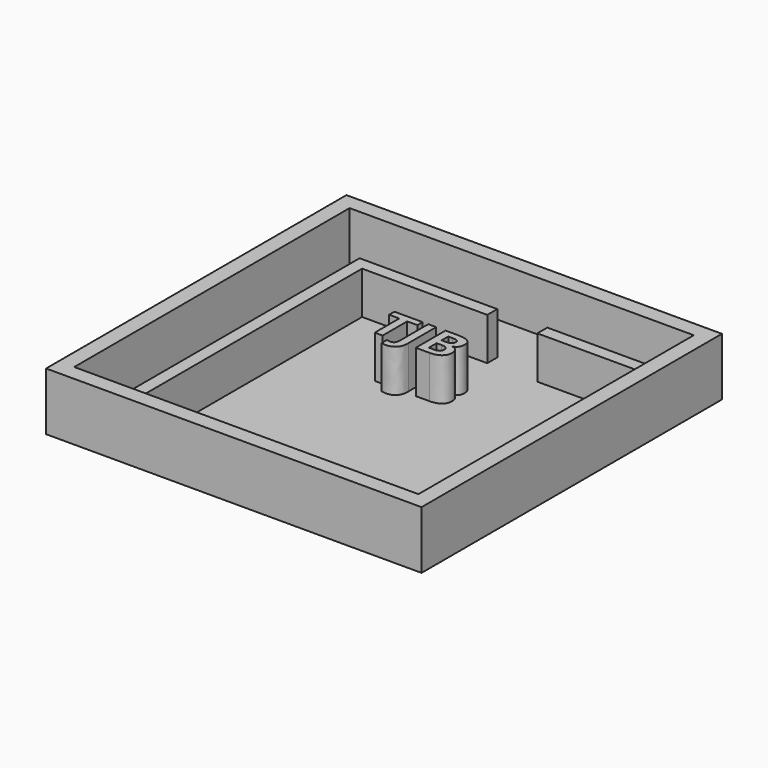
from build123d import *

# Parameters (mm, degrees)
F0_W         = 38.1
F0_H         = 38.1
F1_DEPTH     = 0.79375
F2_W         = 38.1
F2_H         = 38.1
F2_W_2       = 34.925
F2_H_2       = 34.925
F3_DEPTH     = 5.08
F4_W         = 10.795
F4_H         = 1.27
F5_DEPTH     = 4.318
F6_R         = 1.27
F7_DEPTH     = 0.79475
F8_TEXT_SIZE = 5.2916666667
F9_DEPTH     = 4.318


# Not quite as in the source:
# - Text() gives the source's letters only with a copy of the font that has no kerning and outlines rounded to 1/6400 em; it was checked with that copy


with BuildPart() as f1:
    # F0 (on Top) → F1 (new body)
    with BuildSketch(Plane.XY):
        with Locations((33.000832659, -41.2848873556)):
            Rectangle(F0_W, F0_H)
    extrude(amount=F1_DEPTH)

    # F2 (on face) → F3 (join)
    with BuildSketch(Plane.XY.offset(0.79375)):
        with Locations((33.000832659, -41.2848873556)):
            Rectangle(F2_W, F2_H)
        with Locations((33.000832659, -41.2848873556)):
            Rectangle(F2_W_2, F2_H_2, mode=Mode.SUBTRACT)
    extrude(amount=F3_DEPTH)

    # F4 (on face) → F5 (join)
    with BuildSketch(Plane.XY.offset(0.79375)):
        Polygon((20.618332659, -28.9023873556), (20.618332659, -58.7473873556), (21.888332659, -58.7473873556), (21.888332659, -30.1723873556), (34.588332659, -30.1723873556), (34.588332659, -28.9023873556), align=None)
        with Locations((45.065832659, -29.5373873556)):
            Rectangle(F4_W, F4_H)
    extrude(amount=F5_DEPTH)

    # F6 (on face) → F7 (cut, through all)
    with BuildSketch(Plane.XY.offset(0.79375)):
        with Locations((18.0053139994, -56.0103554734)):
            Circle(F6_R)
    extrude(amount=-F7_DEPTH, mode=Mode.SUBTRACT)

    # F8 (on face) → F9 (join)
    with BuildSketch(Plane.XY.offset(0.79375)):
        with Locations((28.3986319387, -38.118737637)):
            Text('TJB', F8_TEXT_SIZE, font='Open Sans', font_style=FontStyle.BOLD, text_align=(TextAlign.LEFT, TextAlign.BOTTOM))
    extrude(amount=F9_DEPTH)


solid = f1.part
